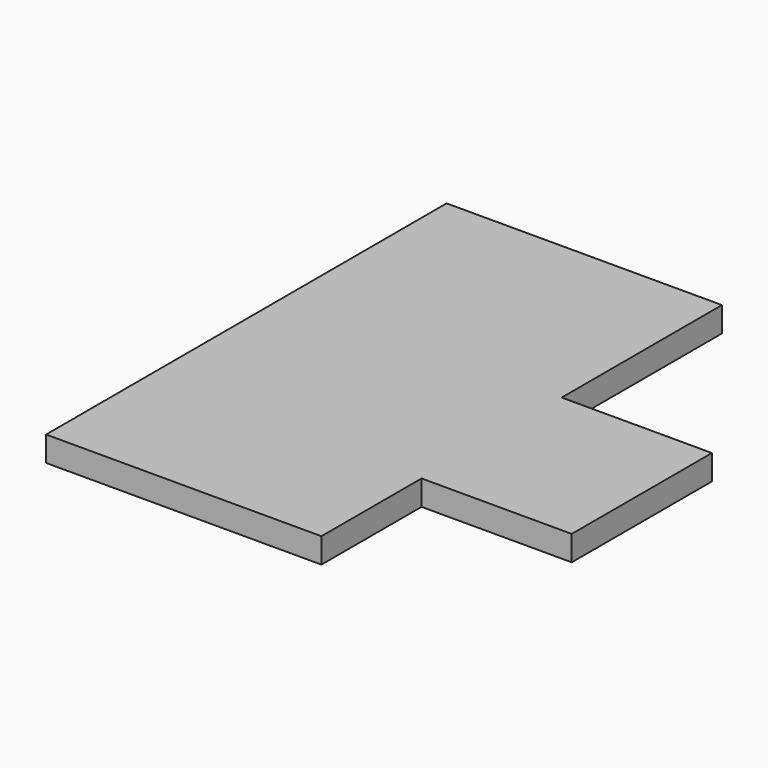
from build123d import *

# Parameters (mm, degrees)
F0_W     = 215.9
F0_H     = 254
F1_DEPTH = 12.7
F3_W     = 76.2
F3_H     = 101.6
F3_H_2   = 63.5
F4_DEPTH = 12.701


with BuildPart() as f1:
    # F0 (on Top) → F1 (new body)
    with BuildSketch(Plane.XY):
        Rectangle(F0_W, F0_H)
    extrude(amount=F1_DEPTH)

    # F3 (on face) → F4 (cut, through all)
    with BuildSketch(Plane.XY.offset(12.7)):
        with Locations((69.85, 76.2)):
            Rectangle(F3_W, F3_H)
        with Locations((69.85, -95.25)):
            Rectangle(F3_W, F3_H_2)
    extrude(amount=-F4_DEPTH, mode=Mode.SUBTRACT)


solid = f1.part
